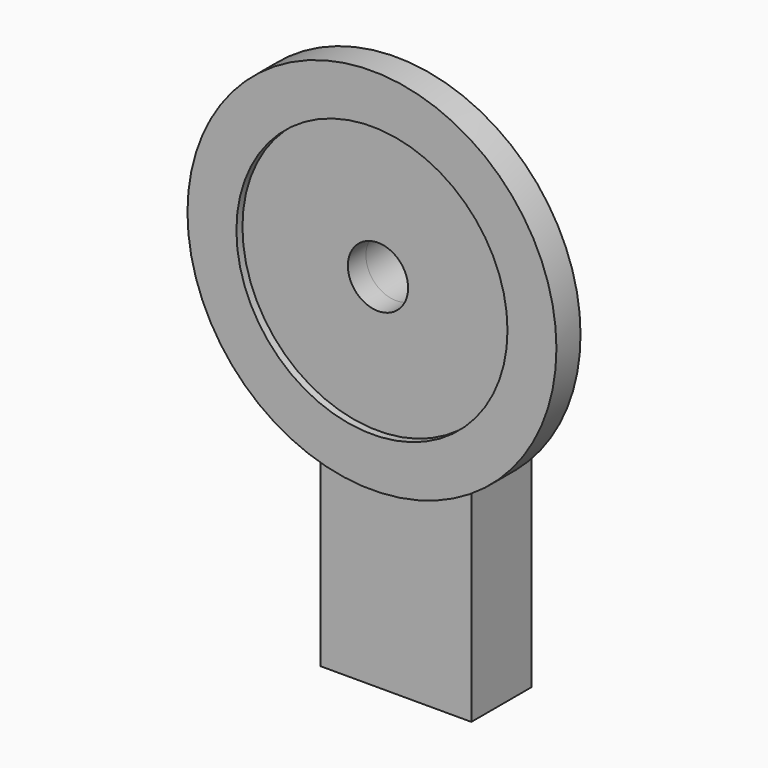
from build123d import *

# Parameters (mm, degrees)
F0_R     = 38.89375
F0_R_2   = 6.35
F1_DEPTH = 4.7625
F2_R     = 38.89375
F2_R_2   = 28.575
F3_DEPTH = 1.5875
F4_R     = 6.35
F5_DEPTH = 15.875
F7_DEPTH = 12.7
F7_TAPER = 5
F8_R     = 3.175
F9_DEPTH = 12.7


with BuildPart() as f1:
    # F0 (on Front) → F1 (new body)
    with BuildSketch(Plane.XZ):
        Circle(F0_R)
        Circle(F0_R_2, mode=Mode.SUBTRACT)
    extrude(amount=F1_DEPTH)

    # F2 (on face) → F3 (join)
    with BuildSketch(Plane.XZ.offset(4.7625)):
        Circle(F2_R)
        Circle(F2_R_2, mode=Mode.SUBTRACT)
    extrude(amount=F3_DEPTH)

    # F4 (on face) → F5 (join)
    with BuildSketch(Plane(origin=(0, 0, 0), x_dir=(-1, 0, 0), z_dir=(0, 1, 0))):
        with BuildLine():
            Line((-15.875, -79.375), (15.875, -79.375))
            Line((15.875, -79.375), (15.875, -35.5064524286))
            ThreePointArc((15.875, -35.5064524286), (0, -38.89375), (-15.875, -35.5064524286))
            Line((-15.875, -35.5064524286), (-15.875, -79.375))
        make_face()
        with BuildLine():
            ThreePointArc((-15.875, -35.5064524286), (0, -38.89375), (15.875, -35.5064524286))
            Line((15.875, -35.5064524286), (15.875, 0))
            ThreePointArc((15.875, 0), (4.9e-09, -15.875), (-15.875, -9.8e-09))
            Line((-15.875, -9.8e-09), (-15.875, -35.5064524286))
        make_face()
        with BuildLine():
            ThreePointArc((-15.875, -9.8e-09), (4.9e-09, -15.875), (15.875, 0))
            ThreePointArc((15.875, 0), (-4.9e-09, 15.875), (-15.875, -9.8e-09))
        make_face()
        Circle(F4_R, mode=Mode.SUBTRACT)
    extrude(amount=F5_DEPTH)

    # F6 (on face) → F7 (cut)
    with BuildSketch(Plane(origin=(0, 15.875, 0), x_dir=(-1, 0, 0), z_dir=(0, 1, 0))):
        with BuildLine():
            ThreePointArc((-6.35, -60.325), (-4.4901280605, -64.8151280605), (0, -66.675))
            Line((0, -66.675), (0, -60.325))
            Line((0, -60.325), (-6.35, -60.325))
        make_face()
        with BuildLine():
            Line((0, -60.325), (0, -66.675))
            ThreePointArc((0, -66.675), (4.4901280605, -64.8151280605), (6.35, -60.325))
            Line((6.35, -60.325), (0, -60.325))
        make_face()
        with BuildLine():
            Line((-6.35, -60.325), (0, -60.325))
            Line((0, -60.325), (0, -53.975))
            ThreePointArc((0, -53.975), (-4.4901280605, -55.8348719395), (-6.35, -60.325))
        make_face()
        with BuildLine():
            Line((0, -53.975), (0, -60.325))
            Line((0, -60.325), (6.35, -60.325))
            ThreePointArc((6.35, -60.325), (4.4901280605, -55.8348719395), (0, -53.975))
        make_face()
        with BuildLine():
            Line((-6.35, -22.225), (-6.35, -60.325))
            ThreePointArc((-6.35, -60.325), (-4.4901280605, -55.8348719395), (0, -53.975))
            Line((0, -53.975), (0, -28.575))
            ThreePointArc((0, -28.575), (-4.4901280605, -26.7151280605), (-6.35, -22.225))
        make_face()
        with BuildLine():
            ThreePointArc((0, -53.975), (4.4901280605, -55.8348719395), (6.35, -60.325))
            Line((6.35, -60.325), (6.35, -22.225))
            ThreePointArc((6.35, -22.225), (4.4901280605, -26.7151280605), (0, -28.575))
            Line((0, -28.575), (0, -53.975))
        make_face()
        with BuildLine():
            ThreePointArc((0, -15.875), (-4.4901280605, -17.7348719395), (-6.35, -22.225))
            Line((-6.35, -22.225), (0, -22.225))
            Line((0, -22.225), (0, -15.875))
        make_face()
        with BuildLine():
            Line((0, -22.225), (-6.35, -22.225))
            ThreePointArc((-6.35, -22.225), (-4.4901280605, -26.7151280605), (0, -28.575))
            Line((0, -28.575), (0, -22.225))
        make_face()
        with BuildLine():
            ThreePointArc((0, -28.575), (4.4901280605, -26.7151280605), (6.35, -22.225))
            Line((6.35, -22.225), (0, -22.225))
            Line((0, -22.225), (0, -28.575))
        make_face()
        with BuildLine():
            Line((0, -22.225), (6.35, -22.225))
            ThreePointArc((6.35, -22.225), (4.4901280605, -17.7348719395), (0, -15.875))
            Line((0, -15.875), (0, -22.225))
        make_face()
    extrude(amount=-F7_DEPTH, taper=F7_TAPER, mode=Mode.SUBTRACT)

    # F8 (on face) → F9 (cut)
    with BuildSketch(Plane(origin=(0, 15.875, 0), x_dir=(-1, 0, 0), z_dir=(0, 1, 0))):
        with BuildLine():
            ThreePointArc((3.175, -11.1125), (2.2450640303, -8.8674359697), (0, -7.9375))
            Line((0, -7.9375), (0, -14.2875))
            ThreePointArc((0, -14.2875), (2.2450640303, -13.3575640303), (3.175, -11.1125))
        make_face()
        with BuildLine():
            ThreePointArc((12.7, -69.85), (9.525, -66.675), (6.35, -69.85))
            ThreePointArc((6.35, -69.85), (9.525, -73.025), (12.7, -69.85))
        make_face()
        with Locations((-9.525, -69.85)):
            Circle(F8_R)
        with BuildLine():
            Line((0, -14.2875), (0, -7.9375))
            ThreePointArc((0, -7.9375), (-3.175, -11.1125), (0, -14.2875))
        make_face()
    extrude(amount=-F9_DEPTH, mode=Mode.SUBTRACT)


solid = f1.part
